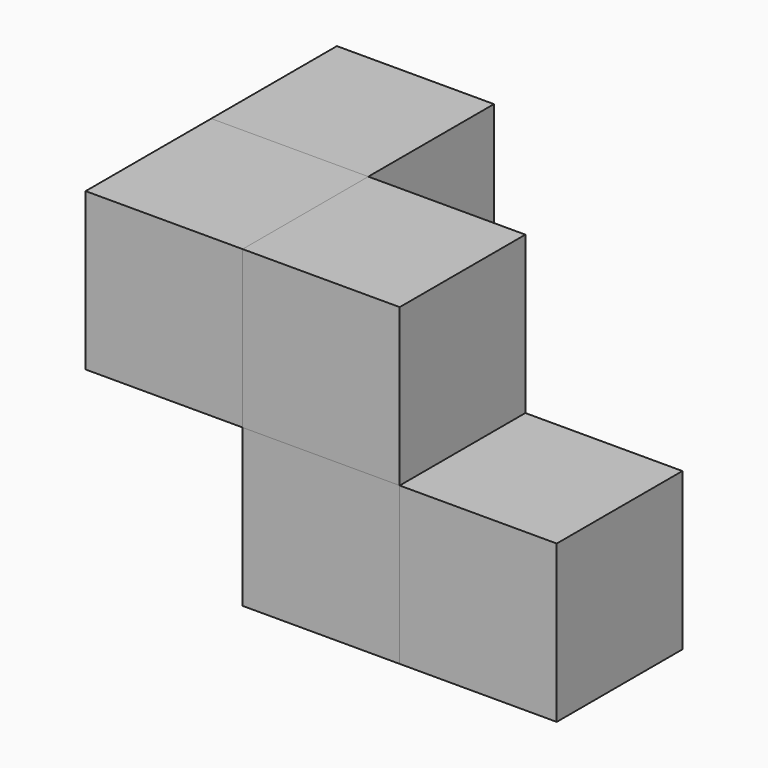
from build123d import *

# Parameters (mm, degrees)
F0_W     = 12.7
F0_H     = 12.7
F1_DEPTH = 12.7


with BuildPart() as f1:
    # F0 (on Front) → F1 (new body)
    with BuildSketch(Plane.XZ):
        with Locations((101.516704464, -3.3304238856)):
            Rectangle(F0_W, F0_H)
    extrude(amount=F1_DEPTH)


with BuildPart() as f2_1:
    # F2: copy of F1
    add(f1.part.moved(Location((12.7, 0, 0))))


with BuildPart() as f3_1:
    # F3: copy of F1
    add(f1.part.moved(Location((0, 0, 12.7))))


with BuildPart() as f6_1:
    # F6: copy of F3_1
    add(f3_1.part.moved(Location((-12.7, 0, 0))))


with BuildPart() as f9_1:
    # F9: copy of F6_1
    add(f6_1.part.moved(Location((0, 12.7, 0))))


solid = Compound([f1.part, f2_1.part, f3_1.part, f6_1.part, f9_1.part])
